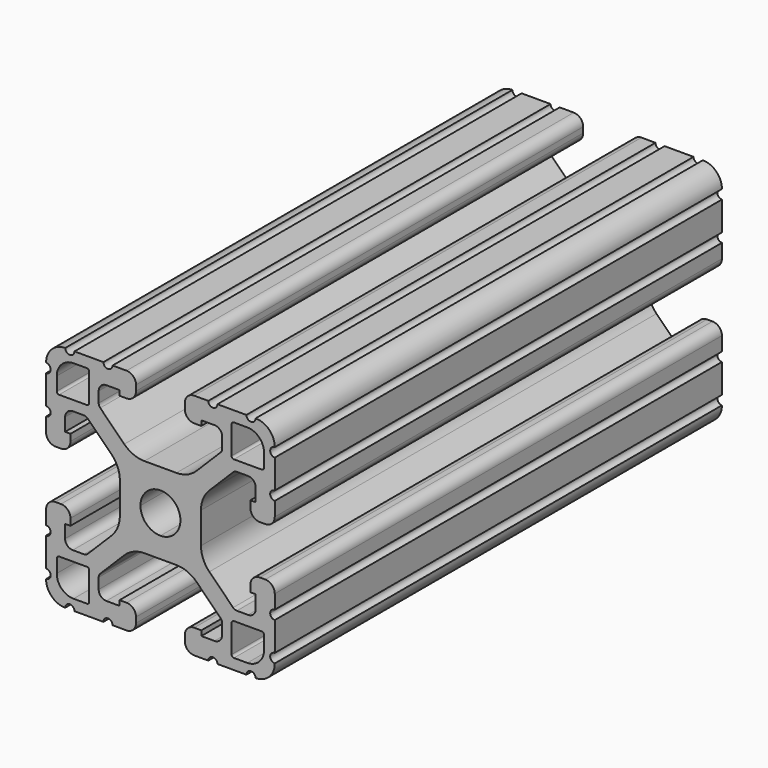
from build123d import *

# Parameters (mm, degrees)
F1_DEPTH = 93.12667


# Not quite as in the source:
# - ends of sketch curves that miss each other by under 0.0002 mm in the source are joined


with BuildPart() as f1:
    # F0 (on Front) → F1 (new body)
    with BuildSketch(Plane.XZ):
        with BuildLine():
            ThreePointArc((-126.395226, 42.8244), (-125.8564106327, 42.6012153673), (-125.633226, 42.0624))
            ThreePointArc((-125.633226, 42.0624), (-125.8564106327, 41.5235846327), (-126.395226, 41.3004))
            Line((-126.395226, 41.3004), (-126.395226, 41.2623))
            Line((-126.395226, 41.2623), (-126.395226, 36.4744))
            ThreePointArc((-126.395226, 36.4744), (-125.6332006, 35.70605), (-126.3952260069, 34.9377008392))
            ThreePointArc((-126.3952260069, 34.9377008392), (-125.4653154303, 32.6799105697), (-123.2075260004, 31.7500001018))
            ThreePointArc((-123.2075260004, 31.7500001018), (-122.439176, 32.5120254), (-121.6708268392, 31.7499999931))
            Line((-121.6708268392, 31.7499999931), (-116.844826, 31.75))
            ThreePointArc((-116.844826, 31.75), (-116.082826, 32.512), (-115.320826, 31.75))
            Line((-115.320826, 31.75), (-112.984026, 31.75))
            ThreePointArc((-112.984026, 31.75), (-111.870474241, 32.211248241), (-111.409226, 33.3248))
            Line((-111.409226, 33.3248), (-111.409226, 34.2392))
            ThreePointArc((-111.409226, 34.2392), (-111.870474241, 35.352751759), (-112.984026, 35.814))
            Line((-112.984026, 35.814), (-114.1593602, 35.814))
            Line((-114.1593602, 35.814), (-114.1593602, 34.975292))
            Line((-114.1593602, 34.975292), (-116.362226, 34.975292))
            ThreePointArc((-116.362226, 34.975292), (-117.2602516121, 35.3472663879), (-117.632226, 36.245292))
            Line((-117.632226, 36.245292), (-117.632226, 38.0197868))
            ThreePointArc((-117.632226, 38.0197868), (-117.5645759596, 38.3598505949), (-117.3719270372, 38.6481322372))
            Line((-117.3719270372, 38.6481322372), (-113.366677, 42.652696))
            ThreePointArc((-113.366677, 42.652696), (-111.8258270387, 43.6821186048), (-110.0083398, 44.0436))
            Line((-110.0083398, 44.0436), (-104.6821122, 44.0436))
            ThreePointArc((-104.6821122, 44.0436), (-102.8646249613, 43.6821186048), (-101.3237758223, 42.6526951776))
            Line((-101.3237758223, 42.6526951776), (-97.3185252, 38.648132))
            ThreePointArc((-97.3185252, 38.648132), (-97.1258760404, 38.3598505949), (-97.058226, 38.0197868))
            Line((-97.058226, 38.0197868), (-97.058226, 36.245292))
            ThreePointArc((-97.058226, 36.245292), (-97.4302003879, 35.3472663879), (-98.328226, 34.975292))
            Line((-98.328226, 34.975292), (-100.5310918, 34.975292))
            Line((-100.5310918, 34.975292), (-100.5310918, 35.814))
            Line((-100.5310918, 35.814), (-101.706426, 35.814))
            ThreePointArc((-101.706426, 35.814), (-102.819977759, 35.352751759), (-103.281226, 34.2392))
            Line((-103.281226, 34.2392), (-103.281226, 33.3248))
            ThreePointArc((-103.281226, 33.3248), (-102.819977759, 32.211248241), (-101.706426, 31.75))
            Line((-101.706426, 31.75), (-99.369626, 31.75))
            ThreePointArc((-99.369626, 31.75), (-98.607626, 32.512), (-97.845626, 31.75))
            Line((-97.845626, 31.75), (-93.019626, 31.75))
            ThreePointArc((-93.019626, 31.75), (-92.251276, 32.5120254), (-91.4829268392, 31.7499999931))
            ThreePointArc((-91.4829268392, 31.7499999931), (-89.2251365697, 32.6799105697), (-88.2952261018, 34.9376999996))
            ThreePointArc((-88.2952261018, 34.9376999996), (-89.0572514, 35.70605), (-88.2952259931, 36.4743991608))
            Line((-88.2952259931, 36.4743991608), (-88.295226, 41.2623))
            Line((-88.295226, 41.2623), (-88.295226, 41.3004))
            ThreePointArc((-88.295226, 41.3004), (-88.8340413673, 41.5235846327), (-89.057226, 42.0624))
            ThreePointArc((-89.057226, 42.0624), (-88.8340413673, 42.6012153673), (-88.295226, 42.8244))
            Line((-88.295226, 42.8244), (-88.295226, 42.8625))
            Line((-88.295226, 42.8625), (-88.295226, 45.1612))
            ThreePointArc((-88.295226, 45.1612), (-88.756474241, 46.274751759), (-89.870026, 46.736))
            Line((-89.870026, 46.736), (-90.784426, 46.736))
            ThreePointArc((-90.784426, 46.736), (-91.897977759, 46.274751759), (-92.359226, 45.1612))
            Line((-92.359226, 45.1612), (-92.359226, 44.0493658))
            Line((-92.359226, 44.0493658), (-91.4661874, 44.0493658))
            Line((-91.4661874, 44.0493658), (-91.4661874, 41.88079))
            ThreePointArc((-91.4661874, 41.88079), (-91.8381617879, 40.9827643879), (-92.7361874, 40.61079))
            Line((-92.7361874, 40.61079), (-94.6024524, 40.61079))
            ThreePointArc((-94.6024524, 40.61079), (-94.9426164872, 40.6784439135), (-95.2310068247, 40.8711085741))
            Line((-95.2310068247, 40.8711085741), (-99.1973632, 44.8367912))
            ThreePointArc((-99.1973632, 44.8367912), (-100.227189958, 46.3778520119), (-100.588826, 48.1957126))
            Line((-100.588826, 48.1957126), (-100.588826, 53.4042874))
            ThreePointArc((-100.588826, 53.4042874), (-100.227189958, 55.2221479881), (-99.1973496778, 56.7631952754))
            Line((-99.1973496778, 56.7631952754), (-95.2310008, 60.7288854))
            ThreePointArc((-95.2310008, 60.7288854), (-94.9426164872, 60.9215560865), (-94.6024524, 60.98921))
            Line((-94.6024524, 60.98921), (-92.7361874, 60.98921))
            ThreePointArc((-92.7361874, 60.98921), (-91.8381617879, 60.6172356121), (-91.4661874, 59.71921))
            Line((-91.4661874, 59.71921), (-91.4661874, 57.5506342))
            Line((-91.4661874, 57.5506342), (-92.359226, 57.5506342))
            Line((-92.359226, 57.5506342), (-92.359226, 56.4388))
            ThreePointArc((-92.359226, 56.4388), (-91.897977759, 55.325248241), (-90.784426, 54.864))
            Line((-90.784426, 54.864), (-89.870026, 54.864))
            ThreePointArc((-89.870026, 54.864), (-88.756474241, 55.325248241), (-88.295226, 56.4388))
            Line((-88.295226, 56.4388), (-88.295226, 58.7375))
            Line((-88.295226, 58.7375), (-88.295226, 58.7756))
            ThreePointArc((-88.295226, 58.7756), (-88.8340413673, 58.9987846327), (-89.057226, 59.5376))
            ThreePointArc((-89.057226, 59.5376), (-88.8340413673, 60.0764153673), (-88.295226, 60.2996))
            Line((-88.295226, 60.2996), (-88.295226, 60.3377))
            Line((-88.295226, 60.3377), (-88.295226, 65.1256))
            ThreePointArc((-88.295226, 65.1256), (-89.0572514, 65.89395), (-88.2952259931, 66.6622991608))
            ThreePointArc((-88.2952259931, 66.6622991608), (-89.2251365697, 68.9200894303), (-91.4829259996, 69.8499998982))
            ThreePointArc((-91.4829259996, 69.8499998982), (-92.251276, 69.0879746), (-93.0196251608, 69.8500000069))
            Line((-93.0196251608, 69.8500000069), (-97.845626, 69.85))
            ThreePointArc((-97.845626, 69.85), (-98.607626, 69.088), (-99.369626, 69.85))
            Line((-99.369626, 69.85), (-101.706426, 69.85))
            ThreePointArc((-101.706426, 69.85), (-102.819977759, 69.388751759), (-103.281226, 68.2752))
            Line((-103.281226, 68.2752), (-103.281226, 67.3608))
            ThreePointArc((-103.281226, 67.3608), (-102.819977759, 66.247248241), (-101.706426, 65.786))
            Line((-101.706426, 65.786), (-100.5310918, 65.786))
            Line((-100.5310918, 65.786), (-100.5310918, 66.624708))
            Line((-100.5310918, 66.624708), (-98.328226, 66.624708))
            ThreePointArc((-98.328226, 66.624708), (-97.4302003879, 66.2527336121), (-97.058226, 65.354708))
            Line((-97.058226, 65.354708), (-97.058226, 63.5802132))
            ThreePointArc((-97.058226, 63.5802132), (-97.1258760404, 63.2401494051), (-97.3185249628, 62.9518677628))
            Line((-97.3185249628, 62.9518677628), (-101.323775, 58.947304))
            ThreePointArc((-101.323775, 58.947304), (-102.8646249613, 57.9178813952), (-104.6821122, 57.5564))
            Line((-104.6821122, 57.5564), (-110.0083398, 57.5564))
            ThreePointArc((-110.0083398, 57.5564), (-111.8258270387, 57.9178813952), (-113.3666761777, 58.9473048224))
            Line((-113.3666761777, 58.9473048224), (-117.3719268, 62.951868))
            ThreePointArc((-117.3719268, 62.951868), (-117.5645759596, 63.2401494051), (-117.632226, 63.5802132))
            Line((-117.632226, 63.5802132), (-117.632226, 65.354708))
            ThreePointArc((-117.632226, 65.354708), (-117.2602516121, 66.2527336121), (-116.362226, 66.624708))
            Line((-116.362226, 66.624708), (-114.1593602, 66.624708))
            Line((-114.1593602, 66.624708), (-114.1593602, 65.786))
            Line((-114.1593602, 65.786), (-112.984026, 65.786))
            ThreePointArc((-112.984026, 65.786), (-111.870474241, 66.247248241), (-111.409226, 67.3608))
            Line((-111.409226, 67.3608), (-111.409226, 68.2752))
            ThreePointArc((-111.409226, 68.2752), (-111.870474241, 69.388751759), (-112.984026, 69.85))
            Line((-112.984026, 69.85), (-115.320826, 69.85))
            ThreePointArc((-115.320826, 69.85), (-116.082826, 69.088), (-116.844826, 69.85))
            Line((-116.844826, 69.85), (-121.670826, 69.85))
            ThreePointArc((-121.670826, 69.85), (-122.439176, 69.0879746), (-123.2075251608, 69.8500000069))
            ThreePointArc((-123.2075251608, 69.8500000069), (-125.4653154303, 68.9200894303), (-126.3952258982, 66.6623000004))
            ThreePointArc((-126.3952258982, 66.6623000004), (-125.6332006, 65.89395), (-126.3952260069, 65.1256008392))
            Line((-126.3952260069, 65.1256008392), (-126.395226, 60.3377))
            Line((-126.395226, 60.3377), (-126.395226, 60.2996))
            ThreePointArc((-126.395226, 60.2996), (-125.8564106327, 60.0764153673), (-125.633226, 59.5376))
            ThreePointArc((-125.633226, 59.5376), (-125.8564106327, 58.9987846327), (-126.395226, 58.7756))
            Line((-126.395226, 58.7756), (-126.395226, 58.7375))
            Line((-126.395226, 58.7375), (-126.395226, 56.4388))
            ThreePointArc((-126.395226, 56.4388), (-125.933977759, 55.325248241), (-124.820426, 54.864))
            Line((-124.820426, 54.864), (-123.906026, 54.864))
            ThreePointArc((-123.906026, 54.864), (-122.792474241, 55.325248241), (-122.331226, 56.4388))
            Line((-122.331226, 56.4388), (-122.331226, 57.5506342))
            Line((-122.331226, 57.5506342), (-123.2242646, 57.5506342))
            Line((-123.2242646, 57.5506342), (-123.2242646, 59.71921))
            ThreePointArc((-123.2242646, 59.71921), (-122.8522902121, 60.6172356121), (-121.9542646, 60.98921))
            Line((-121.9542646, 60.98921), (-120.0879996, 60.98921))
            ThreePointArc((-120.0879996, 60.98921), (-119.7478355128, 60.9215560865), (-119.4594451753, 60.7288914259))
            Line((-119.4594451753, 60.7288914259), (-115.4930888, 56.7632088))
            ThreePointArc((-115.4930888, 56.7632088), (-114.463262042, 55.2221479881), (-114.101626, 53.4042874))
            Line((-114.101626, 53.4042874), (-114.101626, 48.1957126))
            ThreePointArc((-114.101626, 48.1957126), (-114.463262042, 46.3778520119), (-115.4931023222, 44.8368047246))
            Line((-115.4931023222, 44.8368047246), (-119.4594512, 40.8711146))
            ThreePointArc((-119.4594512, 40.8711146), (-119.7478355128, 40.6784439135), (-120.0879996, 40.61079))
            Line((-120.0879996, 40.61079), (-121.9542646, 40.61079))
            ThreePointArc((-121.9542646, 40.61079), (-122.8522902121, 40.9827643879), (-123.2242646, 41.88079))
            Line((-123.2242646, 41.88079), (-123.2242646, 44.0493658))
            Line((-123.2242646, 44.0493658), (-122.331226, 44.0493658))
            Line((-122.331226, 44.0493658), (-122.331226, 45.1612))
            ThreePointArc((-122.331226, 45.1612), (-122.792474241, 46.274751759), (-123.906026, 46.736))
            Line((-123.906026, 46.736), (-124.820426, 46.736))
            ThreePointArc((-124.820426, 46.736), (-125.933977759, 46.274751759), (-126.395226, 45.1612))
            Line((-126.395226, 45.1612), (-126.395226, 42.8625))
            Line((-126.395226, 42.8625), (-126.395226, 42.8244))
        make_face()
        with BuildLine():
            Line((-124.236226, 38.9382), (-119.588026, 38.9382))
            ThreePointArc((-119.588026, 38.9382), (-119.3186183164, 38.8266076836), (-119.207026, 38.5572))
            Line((-119.207026, 38.5572), (-119.207026, 33.909))
            ThreePointArc((-119.207026, 33.909), (-119.3186183164, 33.6395923164), (-119.588026, 33.528))
            Line((-119.588026, 33.528), (-121.823226, 33.528))
            ThreePointArc((-121.823226, 33.528), (-123.7988823466, 34.3463436534), (-124.617226, 36.322))
            Line((-124.617226, 36.322), (-124.617226, 38.5572))
            ThreePointArc((-124.617226, 38.5572), (-124.5056336836, 38.8266076836), (-124.236226, 38.9382))
        make_face(mode=Mode.SUBTRACT)
        with BuildLine():
            Line((-95.102426, 38.9382), (-90.454226, 38.9382))
            ThreePointArc((-90.454226, 38.9382), (-90.1848183164, 38.8266076836), (-90.073226, 38.5572))
            Line((-90.073226, 38.5572), (-90.073226, 36.322))
            ThreePointArc((-90.073226, 36.322), (-90.8915696534, 34.3463436534), (-92.867226, 33.528))
            Line((-92.867226, 33.528), (-95.102426, 33.528))
            ThreePointArc((-95.102426, 33.528), (-95.3718336836, 33.6395923164), (-95.483426, 33.909))
            Line((-95.483426, 33.909), (-95.483426, 38.5572))
            ThreePointArc((-95.483426, 38.5572), (-95.3718336836, 38.8266076836), (-95.102426, 38.9382))
        make_face(mode=Mode.SUBTRACT)
        with BuildLine():
            ThreePointArc((-124.617226, 65.278), (-123.7988823466, 67.2536563466), (-121.823226, 68.072))
            Line((-121.823226, 68.072), (-119.588026, 68.072))
            ThreePointArc((-119.588026, 68.072), (-119.3186183164, 67.9604076836), (-119.207026, 67.691))
            Line((-119.207026, 67.691), (-119.207026, 63.0428))
            ThreePointArc((-119.207026, 63.0428), (-119.3186183164, 62.7733923164), (-119.588026, 62.6618))
            Line((-119.588026, 62.6618), (-124.236226, 62.6618))
            ThreePointArc((-124.236226, 62.6618), (-124.5056336836, 62.7733923164), (-124.617226, 63.0428))
            Line((-124.617226, 63.0428), (-124.617226, 65.278))
        make_face(mode=Mode.SUBTRACT)
        with BuildLine():
            ThreePointArc((-107.345226, 47.4726), (-109.6980531037, 48.4471728963), (-110.672626, 50.8))
            ThreePointArc((-110.672626, 50.8), (-109.6980531037, 53.1528271037), (-107.345226, 54.1274))
            ThreePointArc((-107.345226, 54.1274), (-104.9923988963, 53.1528271037), (-104.017826, 50.8))
            ThreePointArc((-104.017826, 50.8), (-104.9923988963, 48.4471728963), (-107.345226, 47.4726))
        make_face(mode=Mode.SUBTRACT)
        with BuildLine():
            ThreePointArc((-95.483426, 67.691), (-95.3718336836, 67.9604076836), (-95.102426, 68.072))
            Line((-95.102426, 68.072), (-92.867226, 68.072))
            ThreePointArc((-92.867226, 68.072), (-90.8915696534, 67.2536563466), (-90.073226, 65.278))
            Line((-90.073226, 65.278), (-90.073226, 63.0428))
            ThreePointArc((-90.073226, 63.0428), (-90.1848183164, 62.7733923164), (-90.454226, 62.6618))
            Line((-90.454226, 62.6618), (-95.102426, 62.6618))
            ThreePointArc((-95.102426, 62.6618), (-95.3718336836, 62.7733923164), (-95.483426, 63.0428))
            Line((-95.483426, 63.0428), (-95.483426, 67.691))
        make_face(mode=Mode.SUBTRACT)
    extrude(amount=F1_DEPTH)


solid = f1.part
